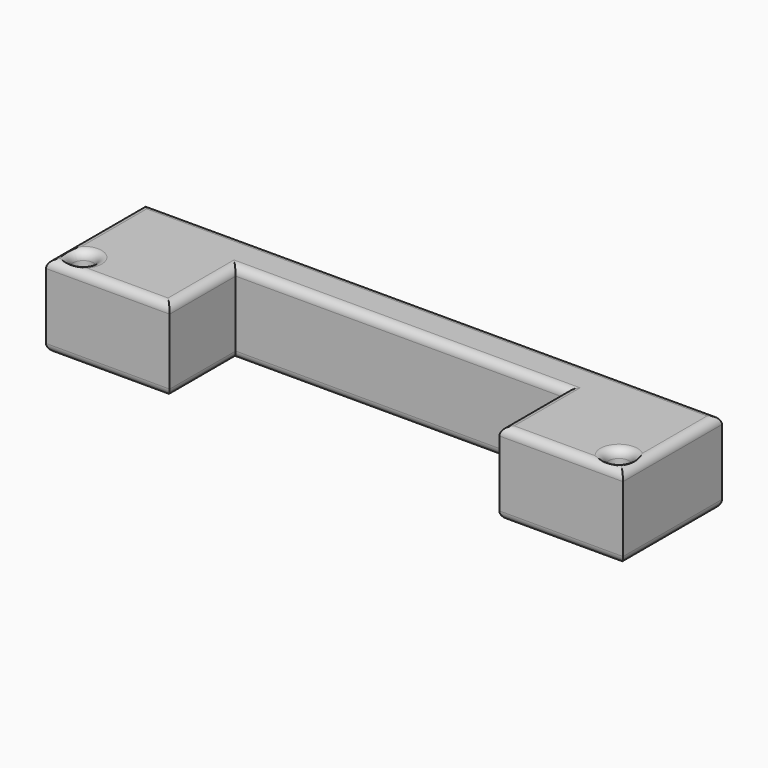
from build123d import *

# Parameters (mm, degrees)
F1_DEPTH     = 20
F3_D         = 5
F5_T1_DEPTH  = 150
F5_T3_DEPTH  = 40
F5_T5_DEPTH  = 40
F5_T7_DEPTH  = 25
F5_T9_DEPTH  = 80
F5_T11_DEPTH = 40
F5_T25_DEPTH = 85
F5_T29_DEPTH = 30
F5_T36_DEPTH = 30
F5_T40_DEPTH = 85
F5_T47_DEPTH = 30
F5_T51_DEPTH = 85
F5_T58_DEPTH = 85
F5_T62_DEPTH = 30


# Not quite as in the source:
# - a fillet or chamfer that OpenCascade refuses, or shapes differently, is made with other operations: its cross-section is extruded or revolved along the edge and cut away or added


with BuildPart() as f1:
    # F0 (on Top) → F1 (new body)
    with BuildSketch(Plane.XY):
        Polygon((70, 32.1153850414), (0, 32.1153850414), (0, 22.1153850414), (40, 22.1153850414), (40, 2.1153850414), (70, 2.1153850414), align=None)
    extrude(amount=F1_DEPTH)

    # F3 (through all)
    with Locations(Plane.XY.offset(20)):
        with Locations((65, 7.1153850414)):
            Hole(F3_D / 2)

    # F4: F1 across face


with BuildPart() as f1_1:
    add(f1.part)
    add(f1.part.mirror(Plane(origin=(0, 27.1153850414, 10), x_dir=(0, -1, 0), z_dir=(-1, 0, 0))))

    # F5: fillet of radius 2 on 20 edges, made by hand

    # F5_s2 → F5_t1 (cut)
    with BuildSketch(Plane.YZ.offset(-75)):
        with BuildLine():
            ThreePointArc((32.1153850414, 18), (31.5295986038, 19.4142135624), (30.1153850414, 20))
            Line((30.1153850414, 20), (32.1153850414, 20))
            Line((32.1153850414, 20), (32.1153850414, 18))
        make_face()
        with BuildLine():
            ThreePointArc((32.1153850414, 2), (31.5295986038, 0.5857864376), (30.1153850414, 0))
            Line((30.1153850414, 0), (32.1153850414, 0))
            Line((32.1153850414, 0), (32.1153850414, 2))
        make_face()
    extrude(amount=F5_T1_DEPTH, mode=Mode.SUBTRACT)

    # F5_s4 → F5_t3 (cut)
    with BuildSketch(Plane.XZ.offset(-37.1153850414)):
        with BuildLine():
            ThreePointArc((-70, 18), (-69.4142135624, 19.4142135624), (-68, 20))
            Line((-68, 20), (-70, 20))
            Line((-70, 20), (-70, 18))
        make_face()
        with BuildLine():
            ThreePointArc((68, 20), (69.4142135624, 19.4142135624), (70, 18))
            Line((70, 18), (70, 20))
            Line((70, 20), (68, 20))
        make_face()
        with BuildLine():
            ThreePointArc((-68, 0), (-69.4142135624, 0.5857864376), (-70, 2))
            Line((-70, 2), (-70, 0))
            Line((-70, 0), (-68, 0))
        make_face()
        with BuildLine():
            ThreePointArc((68, 0), (69.4142135624, 0.5857864376), (70, 2))
            Line((70, 2), (70, 0))
            Line((70, 0), (68, 0))
        make_face()
    extrude(amount=F5_T3_DEPTH, mode=Mode.SUBTRACT)

    # F5_s6 → F5_t5 (cut)
    with BuildSketch(Plane.YZ.offset(-75)):
        with BuildLine():
            ThreePointArc((2.1153850414, 18), (2.701171479, 19.4142135624), (4.1153850414, 20))
            Line((4.1153850414, 20), (2.1153850414, 20))
            Line((2.1153850414, 20), (2.1153850414, 18))
        make_face()
        with BuildLine():
            ThreePointArc((4.1153850414, 0), (2.701171479, 0.5857864376), (2.1153850414, 2))
            Line((2.1153850414, 2), (2.1153850414, 0))
            Line((2.1153850414, 0), (4.1153850414, 0))
        make_face()
    extrude(amount=F5_T5_DEPTH, mode=Mode.SUBTRACT)

    # F5_s8 → F5_t7 (cut)
    with BuildSketch(Plane.XZ.offset(-22.1153850414)):
        with BuildLine():
            ThreePointArc((-40, 18), (-40.5857864376, 19.4142135624), (-42, 20))
            Line((-42, 20), (-40, 20))
            Line((-40, 20), (-40, 18))
        make_face()
        with BuildLine():
            ThreePointArc((40, 18), (40.5857864376, 19.4142135624), (42, 20))
            Line((42, 20), (40, 20))
            Line((40, 20), (40, 18))
        make_face()
        with BuildLine():
            ThreePointArc((-42, 0), (-40.5857864376, 0.5857864376), (-40, 2))
            Line((-40, 2), (-40, 0))
            Line((-40, 0), (-42, 0))
        make_face()
        with BuildLine():
            ThreePointArc((42, 0), (40.5857864376, 0.5857864376), (40, 2))
            Line((40, 2), (40, 0))
            Line((40, 0), (42, 0))
        make_face()
    extrude(amount=F5_T7_DEPTH, mode=Mode.SUBTRACT)

    # F5_s10 → F5_t9 (cut)
    with BuildSketch(Plane.YZ.offset(-40)):
        with BuildLine():
            ThreePointArc((22.1153850414, 18), (22.701171479, 19.4142135624), (24.1153850414, 20))
            Line((24.1153850414, 20), (22.1153850414, 20))
            Line((22.1153850414, 20), (22.1153850414, 18))
        make_face()
        with BuildLine():
            ThreePointArc((24.1153850414, 0), (22.701171479, 0.5857864376), (22.1153850414, 2))
            Line((22.1153850414, 2), (22.1153850414, 0))
            Line((22.1153850414, 0), (24.1153850414, 0))
        make_face()
    extrude(amount=F5_T9_DEPTH, mode=Mode.SUBTRACT)

    # F5_s12 → F5_t11 (cut)
    with BuildSketch(Plane.YZ.offset(35)):
        with BuildLine():
            ThreePointArc((2.1153850414, 18), (2.701171479, 19.4142135624), (4.1153850414, 20))
            Line((4.1153850414, 20), (2.1153850414, 20))
            Line((2.1153850414, 20), (2.1153850414, 18))
        make_face()
        with BuildLine():
            ThreePointArc((4.1153850414, 0), (2.701171479, 0.5857864376), (2.1153850414, 2))
            Line((2.1153850414, 2), (2.1153850414, 0))
            Line((2.1153850414, 0), (4.1153850414, 0))
        make_face()
    extrude(amount=F5_T11_DEPTH, mode=Mode.SUBTRACT)

    # F5_s13 → F5_t14 (revolve, cut)
    with BuildSketch(Plane.XZ.offset(-7.1153850414)):
        with BuildLine():
            ThreePointArc((67.5, 18), (68.0857864376, 19.4142135624), (69.5, 20))
            Line((69.5, 20), (67.5, 20))
            Line((67.5, 20), (67.5, 18))
        make_face()
    revolve(axis=Axis((65, 7.1153850414, 20), (0, 0, 1)), mode=Mode.SUBTRACT)

    # F5_s15 → F5_t16 (revolve, cut)
    with BuildSketch(Plane.XZ.offset(-7.1153850414)):
        with BuildLine():
            ThreePointArc((-67.5, 18), (-68.0857864376, 19.4142135624), (-69.5, 20))
            Line((-69.5, 20), (-67.5, 20))
            Line((-67.5, 20), (-67.5, 18))
        make_face()
    revolve(axis=Axis((-65, 7.1153850414, 20), (0, 0, -1)), mode=Mode.SUBTRACT)

    # F5_s17 → F5_t18 (revolve, cut)
    with BuildSketch(Plane.XZ.offset(-7.1153850414)):
        with BuildLine():
            ThreePointArc((69.5, 0), (68.0857864376, 0.5857864376), (67.5, 2))
            Line((67.5, 2), (67.5, 0))
            Line((67.5, 0), (69.5, 0))
        make_face()
    revolve(axis=Axis((65, 7.1153850414, 0), (0, 0, 1)), mode=Mode.SUBTRACT)

    # F5_s19 → F5_t20 (revolve, cut)
    with BuildSketch(Plane.XZ.offset(-7.1153850414)):
        with BuildLine():
            ThreePointArc((-69.5, 0), (-68.0857864376, 0.5857864376), (-67.5, 2))
            Line((-67.5, 2), (-67.5, 0))
            Line((-67.5, 0), (-69.5, 0))
        make_face()
    revolve(axis=Axis((-65, 7.1153850414, 0), (0, 0, -1)), mode=Mode.SUBTRACT)


with BuildPart() as f5_tool23:
    # F5_s24 → F5_t25 (new body)
    with BuildSketch(Plane.YZ.offset(-45)):
        with BuildLine():
            ThreePointArc((22.1153850414, 18), (22.701171479, 19.4142135624), (24.1153850414, 20))
            Line((24.1153850414, 20), (22.1153850414, 20))
            Line((22.1153850414, 20), (22.1153850414, 18))
        make_face()
    extrude(amount=F5_T25_DEPTH)

    split(bisect_by=Plane.YZ.offset(-40), keep=Keep.BOTTOM)


with BuildPart() as f5_tool27:
    # F5_s28 → F5_t29 (new body)
    with BuildSketch(Plane.XZ.offset(-27.1153850414)):
        with BuildLine():
            ThreePointArc((-40, 18), (-40.5857864376, 19.4142135624), (-42, 20))
            Line((-42, 20), (-40, 20))
            Line((-40, 20), (-40, 18))
        make_face()
    extrude(amount=F5_T29_DEPTH)

    split(bisect_by=Plane.XZ.offset(-22.1153850414), keep=Keep.BOTTOM)


with BuildPart() as f5_tool23_1:
    add(f5_tool23.part)

    # F5_t31: intersect F5_tool27
    add(f5_tool27.part, mode=Mode.INTERSECT)


with BuildPart() as f1_2:
    add(f1_1.part)

    # F5_t21: cut F5_tool23
    add(f5_tool23_1.part, mode=Mode.SUBTRACT)


with BuildPart() as f5_tool34:
    # F5_s35 → F5_t36 (new body)
    with BuildSketch(Plane.XZ.offset(-27.1153850414)):
        with BuildLine():
            ThreePointArc((40, 18), (40.5857864376, 19.4142135624), (42, 20))
            Line((42, 20), (40, 20))
            Line((40, 20), (40, 18))
        make_face()
    extrude(amount=F5_T36_DEPTH)

    split(bisect_by=Plane.XZ.offset(-22.1153850414), keep=Keep.BOTTOM)


with BuildPart() as f5_tool38:
    # F5_s39 → F5_t40 (new body)
    with BuildSketch(Plane.YZ.offset(-40)):
        with BuildLine():
            ThreePointArc((22.1153850414, 18), (22.701171479, 19.4142135624), (24.1153850414, 20))
            Line((24.1153850414, 20), (22.1153850414, 20))
            Line((22.1153850414, 20), (22.1153850414, 18))
        make_face()
    extrude(amount=F5_T40_DEPTH)

    split(bisect_by=Plane.YZ.offset(40), keep=Keep.TOP)


with BuildPart() as f5_tool34_1:
    add(f5_tool34.part)

    # F5_t42: intersect F5_tool38
    add(f5_tool38.part, mode=Mode.INTERSECT)


with BuildPart() as f1_3:
    add(f1_2.part)

    # F5_t32: cut F5_tool34
    add(f5_tool34_1.part, mode=Mode.SUBTRACT)


with BuildPart() as f5_tool45:
    # F5_s46 → F5_t47 (new body)
    with BuildSketch(Plane.XZ.offset(-27.1153850414)):
        with BuildLine():
            ThreePointArc((-42, 0), (-40.5857864376, 0.5857864376), (-40, 2))
            Line((-40, 2), (-40, 0))
            Line((-40, 0), (-42, 0))
        make_face()
    extrude(amount=F5_T47_DEPTH)

    split(bisect_by=Plane.XZ.offset(-22.1153850414), keep=Keep.BOTTOM)


with BuildPart() as f5_tool49:
    # F5_s50 → F5_t51 (new body)
    with BuildSketch(Plane.YZ.offset(40)):
        with BuildLine():
            ThreePointArc((24.1153850414, 0), (22.701171479, 0.5857864376), (22.1153850414, 2))
            Line((22.1153850414, 2), (22.1153850414, 0))
            Line((22.1153850414, 0), (24.1153850414, 0))
        make_face()
    extrude(amount=-F5_T51_DEPTH)

    split(bisect_by=Plane.YZ.offset(-40), keep=Keep.BOTTOM)


with BuildPart() as f5_tool45_1:
    add(f5_tool45.part)

    # F5_t53: intersect F5_tool49
    add(f5_tool49.part, mode=Mode.INTERSECT)


with BuildPart() as f1_4:
    add(f1_3.part)

    # F5_t43: cut F5_tool45
    add(f5_tool45_1.part, mode=Mode.SUBTRACT)


with BuildPart() as f5_tool56:
    # F5_s57 → F5_t58 (new body)
    with BuildSketch(Plane.YZ.offset(45)):
        with BuildLine():
            ThreePointArc((24.1153850414, 0), (22.701171479, 0.5857864376), (22.1153850414, 2))
            Line((22.1153850414, 2), (22.1153850414, 0))
            Line((22.1153850414, 0), (24.1153850414, 0))
        make_face()
    extrude(amount=-F5_T58_DEPTH)

    split(bisect_by=Plane.YZ.offset(40), keep=Keep.TOP)


with BuildPart() as f5_tool60:
    # F5_s61 → F5_t62 (new body)
    with BuildSketch(Plane.XZ.offset(-27.1153850414)):
        with BuildLine():
            ThreePointArc((42, 0), (40.5857864376, 0.5857864376), (40, 2))
            Line((40, 2), (40, 0))
            Line((40, 0), (42, 0))
        make_face()
    extrude(amount=F5_T62_DEPTH)

    split(bisect_by=Plane.XZ.offset(-22.1153850414), keep=Keep.BOTTOM)


with BuildPart() as f5_tool56_1:
    add(f5_tool56.part)

    # F5_t64: intersect F5_tool60
    add(f5_tool60.part, mode=Mode.INTERSECT)


with BuildPart() as f1_5:
    add(f1_4.part)

    # F5_t54: cut F5_tool56
    add(f5_tool56_1.part, mode=Mode.SUBTRACT)


solid = f1_5.part
